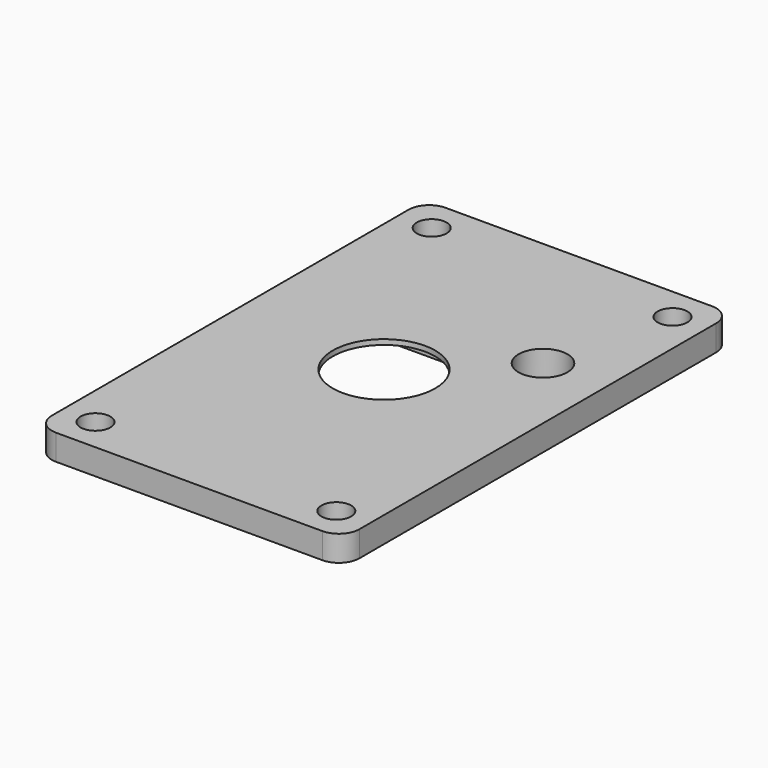
from build123d import *

# Parameters (mm, degrees)
F0_W     = 76.2
F0_H     = 120.65
F0_R     = 3.683
F0_R_2   = 12.7
F0_R_3   = 6.0579
F1_DEPTH = 6.35
F2_R     = 5.08
F3_R     = 12.7
F4_DEPTH = 5.08


# Not quite as in the source:
# - a length typed as a fraction of an inch, garbled in the dataset ("3 / 203.2 mm" for 3/8 in), is restored


with BuildPart() as f1:
    # F0 (on Top) → F1 (new body)
    with BuildSketch(Plane.XY):
        Rectangle(F0_W, F0_H)
        with Locations((-29.8323, -52.0573)):
            Circle(F0_R, mode=Mode.SUBTRACT)
        with Locations((29.8323, -52.0573)):
            Circle(F0_R, mode=Mode.SUBTRACT)
        with Locations((-29.8323, 52.0573)):
            Circle(F0_R, mode=Mode.SUBTRACT)
        Circle(F0_R_2, mode=Mode.SUBTRACT)
        with Locations((22.3901, 21.2471)):
            Circle(F0_R_3, mode=Mode.SUBTRACT)
        with Locations((29.8323, 52.0573)):
            Circle(F0_R, mode=Mode.SUBTRACT)
    extrude(amount=F1_DEPTH)

    # F2
    f2_edges = [f1.edges().sort_by_distance(p)[0] for p in [
        (38.1, -60.325, 3.175),
        (-38.1, 60.325, 3.175),
        (38.1, 60.325, 3.175),
        (-38.1, -60.325, 3.175),
    ]]
    fillet(f2_edges, radius=F2_R)

    # F3 (on face) → F4 (cut)
    with BuildSketch(Plane(origin=(0, 0, 0), x_dir=(1, 0, 0), z_dir=(0, 0, -1))):
        with BuildLine():
            Line((22.86, 19.05), (14.4386043259, 19.05))
            Line((14.4386043259, 19.05), (-22.86, 19.05))
            Line((-22.86, 19.05), (-22.86, -19.05))
            Line((-22.86, -19.05), (13.4802116102, -19.05))
            ThreePointArc((13.4802116102, -19.05), (16.6474146742, -12.7797644882), (22.86, -9.5009213703))
            Line((22.86, -9.5009213703), (22.86, 19.05))
        make_face()
        Circle(F3_R, mode=Mode.SUBTRACT)
    extrude(amount=-F4_DEPTH, mode=Mode.SUBTRACT)


solid = f1.part
